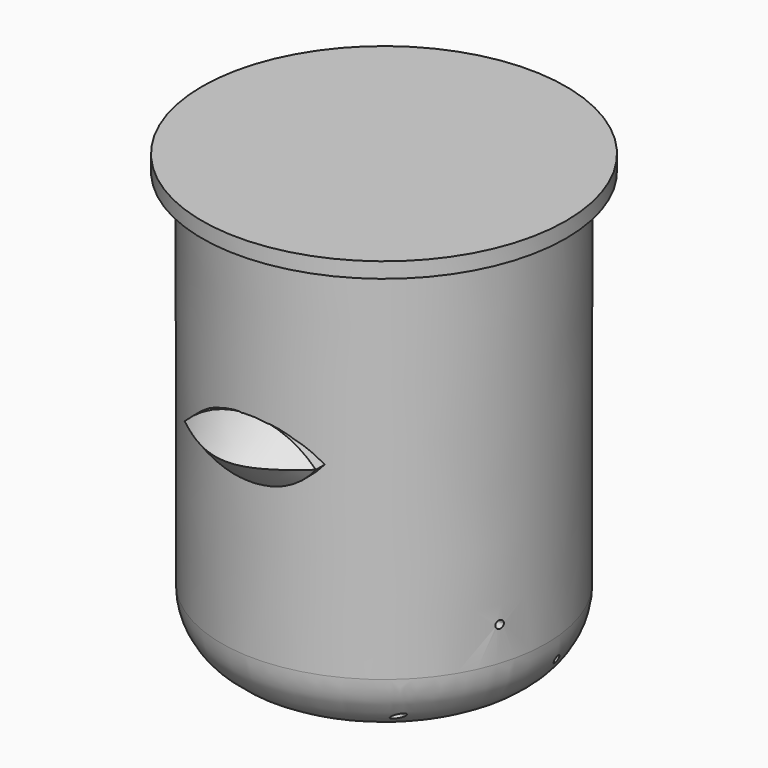
from build123d import *

# Parameters (mm, degrees)
F1_R        = 21.0469324254
F2_R        = 21.1604882825
F4_R        = 8
F7_DEPTH    = 5
F8_SIZE2    = 5
F8_SIZE     = 5
F9_T2_ANGLE = 186.5608570094
F10_R       = 23.5817916237
F11_DEPTH   = 2
F13_R       = 19
F14_DEPTH   = 35
F17_DEPTH   = 58.0661
F19_DEPTH   = 70
F21_DEPTH   = 29.94265


# Not quite as in the source:
# - a fillet or chamfer that OpenCascade refuses, or shapes differently, is made with other operations: its cross-section is extruded or revolved along the edge and cut away or added


with BuildPart() as f3:
    # F1 (on Top) → F3 section 0
    with BuildSketch(Plane.XY):
        Circle(F1_R)
    # F2 (on offset) → F3 section 1
    with BuildSketch(Plane.XY.offset(55)):
        Circle(F2_R)
    loft()

    # F4
    f4_edges = [f3.edges().sort_by_distance(p)[0] for p in [
        (-21.046932, 0, 0),
    ]]
    fillet(f4_edges, radius=F4_R)

    # F13 (on offset) → F14 (cut)
    with BuildSketch(Plane.XY.offset(57)):
        Circle(F13_R)
    extrude(amount=-F14_DEPTH, mode=Mode.SUBTRACT)

    # F16 (on offset) → F17 (cut)
    with BuildSketch(Plane.YZ.offset(21)):
        with BuildLine():
            ThreePointArc((2.6627810146, 4.3431584433), (3.0163344052, 4.4896050527), (3.1627810146, 4.8431584433))
            ThreePointArc((3.1627810146, 4.8431584433), (2.309227624, 5.1967118339), (2.6627810146, 4.3431584433))
        make_face()
    extrude(amount=-F17_DEPTH, mode=Mode.SUBTRACT)

    # F18 (on offset) → F19 (cut)
    with BuildSketch(Plane.YZ.offset(21)):
        with BuildLine():
            ThreePointArc((-13.9506678134, 3.2588179801), (-14.304221204, 2.4052645895), (-13.4506678134, 2.7588179801))
            ThreePointArc((-13.4506678134, 2.7588179801), (-13.5971144228, 3.1123713707), (-13.9506678134, 3.2588179801))
        make_face()
    extrude(amount=-F19_DEPTH, mode=Mode.SUBTRACT)

    # F20 (on offset) → F21 (cut)
    with BuildSketch(Plane.YZ.offset(21)):
        with BuildLine():
            ThreePointArc((-6.3749403842, 11.9251514375), (-6.0213869936, 12.0715980469), (-5.8749403842, 12.4251514375))
            ThreePointArc((-5.8749403842, 12.4251514375), (-6.7284937748, 12.7787048281), (-6.3749403842, 11.9251514375))
        make_face()
    extrude(amount=-F21_DEPTH, mode=Mode.SUBTRACT)


with BuildPart() as f7:
    # F6 (on offset) → F7 (new body, symmetric)
    with BuildSketch(Plane.XZ.offset(21)):
        with BuildLine():
            ThreePointArc((0, 27.9479043256), (4.435903154, 29.1470291114), (7.9694277323, 32.0846031273))
            ThreePointArc((7.9694277323, 32.0846031273), (-0.5305722677, 35.6169163952), (-9.0305722677, 32.0846031273))
            ThreePointArc((-9.0305722677, 32.0846031273), (-5.0201172156, 28.9141880975), (0, 27.9479043256))
        make_face()
    extrude(amount=F7_DEPTH, both=True)

    # F8
    f8_edges = [f7.edges().sort_by_distance(p)[0] for p in [
        (-0.530572, -26, 35.616916),
    ]]
    chamfer(f8_edges, length=F8_SIZE, length2=F8_SIZE2)

    # F9: chamfer of 5 on 1 edges, made by hand

    # F9_s1 → F9_t2 (revolve, cut)
    with BuildSketch(Plane(origin=(-2.2134979331, 0, 38.6185769281), x_dir=(0, 1, 0), z_dir=(-0.057223003, 0, 0.9983614215))):
        Polygon((-21, -12.4658851029), (-26, -7.4658851029), (-26, -12.4658851029), align=None)
    revolve(axis=Axis((-0.5305722677, -26, 38.7150370459), (0, 1, 0)), revolution_arc=F9_T2_ANGLE, mode=Mode.SUBTRACT)


with BuildPart() as f11:
    # F10 (on offset) → F11 (new body)
    with BuildSketch(Plane.XY.offset(55)):
        Circle(F10_R)
    extrude(amount=F11_DEPTH)


solid = Compound([f3.part, f7.part, f11.part])
